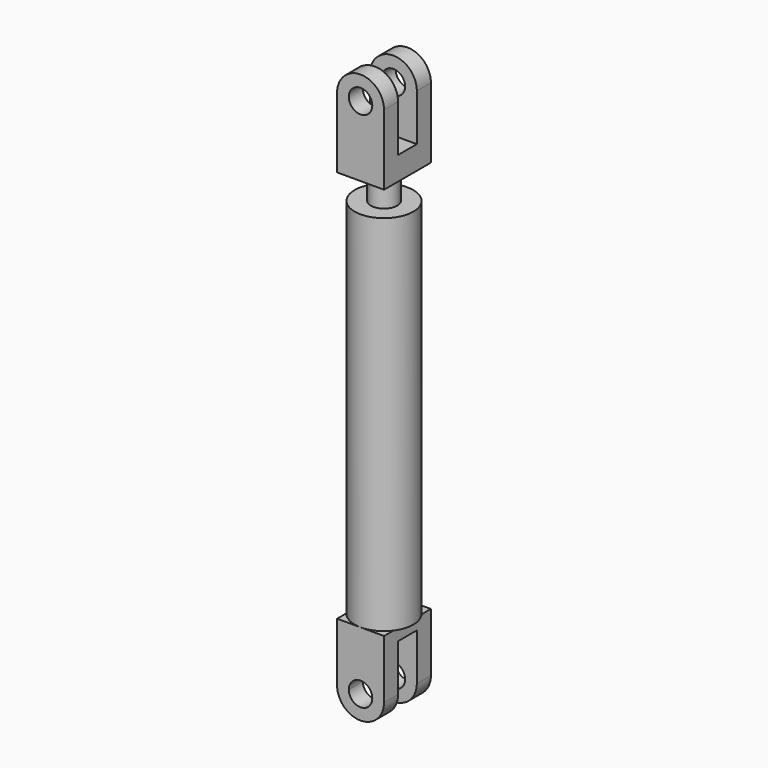
from build123d import *

# Parameters (mm, degrees)
F0_W          = 14.2875
F0_H          = 19.05
F0_W_2        = 11.1125
F3_DEPTH      = 31.75
F4_DEPTH      = 31.75
F7_W          = 25.4
F7_H          = 76.2
F8_DEPTH      = 31.751
F8_DEPTH_BACK = 31.751


with BuildPart() as f1:
    # F0 (on Front) → F1 (revolve)
    with BuildSketch(Plane.XZ):
        Polygon((-25.4, 88.9), (0, 88.9), (0, 488.95), (-14.2875, 488.95), (-14.2875, 457.2), (-14.2875, 431.8), (-14.2875, 127), (-25.4, 127), align=None)
    revolve(axis=Axis((0, 0, 282.575), (0, 0, 1)))

    # F0 (on Front) → F3 (join, symmetric)
    with BuildSketch(Plane.XZ):
        with Locations((-7.14375, 498.475)):
            Rectangle(F0_W, F0_H)
        with Locations((-19.84375, 498.475)):
            Rectangle(F0_W_2, F0_H)
        with BuildLine():
            Line((-14.2875, 508), (0, 508))
            Line((0, 508), (0, 539.75))
            ThreePointArc((0, 539.75), (-7.4747395874, 540.8747395874), (-14.2875, 544.1493489684))
            Line((-14.2875, 544.1493489684), (-14.2875, 508))
        make_face()
        with BuildLine():
            Line((-25.4, 508), (-14.2875, 508))
            Line((-14.2875, 508), (-14.2875, 544.1493489684))
            ThreePointArc((-14.2875, 544.1493489684), (-22.4506403027, 553.270237797), (-25.4, 565.15))
            Line((-25.4, 565.15), (-25.4, 508))
        make_face()
        with BuildLine():
            ThreePointArc((-14.2875, 544.1493489684), (-7.4747395874, 540.8747395874), (0, 539.75))
            ThreePointArc((0, 539.75), (7.4747395874, 540.8747395874), (14.2875, 544.1493489684))
            ThreePointArc((14.2875, 544.1493489684), (22.4506403027, 553.270237797), (25.4, 565.15))
            ThreePointArc((25.4, 565.15), (0, 590.55), (-25.4, 565.15))
            ThreePointArc((-25.4, 565.15), (-22.4506403027, 553.270237797), (-14.2875, 544.1493489684))
        make_face()
        with BuildLine():
            ThreePointArc((12.7, 565.15), (8.9802561211, 556.1697438789), (0, 552.45))
            ThreePointArc((0, 552.45), (-8.9802561211, 574.1302561211), (12.7, 565.15))
        make_face(mode=Mode.SUBTRACT)
    extrude(amount=F3_DEPTH, both=True)

    # F5: F1 across plane


with BuildPart() as f2:
    # F0 (on Front) → F2 (revolve)
    with BuildSketch(Plane.XZ):
        Polygon((-25.4, 63.5), (0, 63.5), (0, 88.9), (-25.4, 88.9), (-25.4, 127), (-25.4, 431.8), (-14.2875, 431.8), (-14.2875, 457.2), (-31.75, 457.2), (-31.75, 63.5), align=None)
    revolve(axis=Axis((0, 0, 282.575), (0, 0, 1)))

    # F0 (on Front) → F4 (join, symmetric)
    with BuildSketch(Plane.XZ):
        with BuildLine():
            ThreePointArc((25.4, 0), (17.9605122421, 17.9605122421), (0, 25.4))
            ThreePointArc((0, 25.4), (-17.9605122421, 17.9605122421), (-25.4, 0))
            ThreePointArc((-25.4, 0), (0, -25.4), (25.4, 0))
        make_face()
        with BuildLine():
            ThreePointArc((0, 12.7), (8.9802561211, 8.9802561211), (12.7, 0))
            ThreePointArc((12.7, 0), (-8.9802561211, -8.9802561211), (0, 12.7))
        make_face(mode=Mode.SUBTRACT)
        with BuildLine():
            ThreePointArc((-25.4, 0), (-17.9605122421, 17.9605122421), (0, 25.4))
            Line((0, 25.4), (0, 63.5))
            Line((0, 63.5), (-25.4, 63.5))
            Line((-25.4, 63.5), (-25.4, 0))
        make_face()
    extrude(amount=F4_DEPTH, both=True)

    # F6: F2 across plane


with BuildPart() as f1_1:
    add(f1.part)
    add(f1.part.mirror(Plane.YZ))


with BuildPart() as f2_1:
    add(f2.part)
    add(f2.part.mirror(Plane.YZ))


with BuildPart() as f8_tool:
    # F7 (on Right) → F8 (new body, two sides)
    with BuildSketch(Plane.YZ) as f8_sk:
        with Locations((0, 552.45)):
            Rectangle(F7_W, F7_H)
        with Locations((0, 12.7)):
            Rectangle(F7_W, F7_H)
    extrude(amount=-F8_DEPTH)
    extrude(f8_sk.sketch, amount=F8_DEPTH_BACK)


with BuildPart() as f1_2:
    add(f1_1.part)

    # F8: cut by f8_tool
    add(f8_tool.part, mode=Mode.SUBTRACT)


with BuildPart() as f2_2:
    add(f2_1.part)

    # F8: cut by f8_tool
    add(f8_tool.part, mode=Mode.SUBTRACT)


solid = Compound([f1_2.part, f2_2.part])
